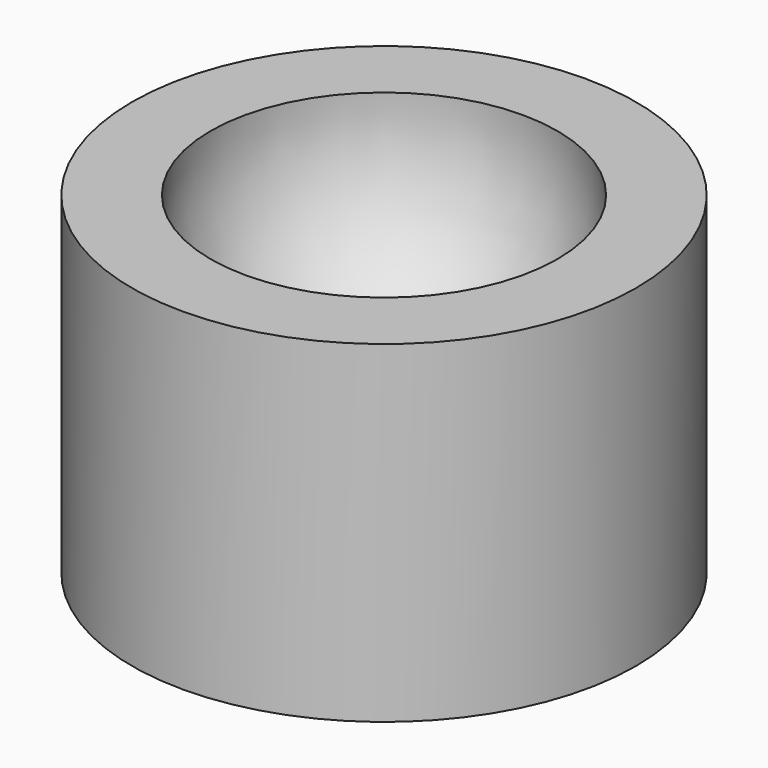
from build123d import *

# Parameters (mm, degrees)
F3_D           = 6.35
F3_CSINK_D     = 12.7
F3_CSINK_ANGLE = 90


# Not quite as in the source:
# - a feature names something its author has since deleted; it is built from what else it names


with BuildPart() as f1:
    # F0 (on Front) → F1 (revolve)
    with BuildSketch(Plane.XZ):
        with BuildLine():
            ThreePointArc((0, -11.2485876307), (-7.1355577219, -8.0776066744), (-9.5645654699, -0.6566077129))
            Line((-9.5645654699, -0.6566077129), (-13.8944359496, -0.6566077129))
            Line((-13.8944359496, -0.6566077129), (-13.8944359496, -19.0012976527))
            Line((-13.8944359496, -19.0012976527), (0, -19.0012976527))
            Line((0, -19.0012976527), (0, -11.2485876307))
        make_face()
    revolve(axis=Axis((0, 0, -15.1249426417), (0, 0, -1)))

    # F3 (through all)
    with Locations(Plane.XY):
        with Locations((0, 0)):
            CounterSinkHole(F3_D / 2, F3_CSINK_D / 2, counter_sink_angle=F3_CSINK_ANGLE)


solid = f1.part
